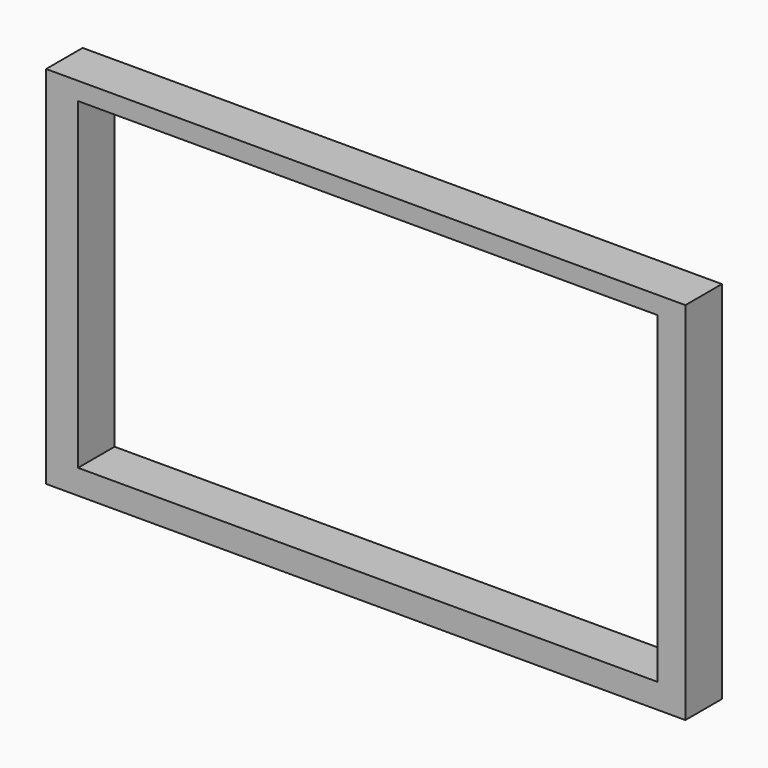
from build123d import *

# Parameters (mm, degrees)
F0_W     = 88.9
F0_H     = 50.8
F0_W_2   = 80.5856101215
F0_H_2   = 44.8976987973
F1_DEPTH = 6.35


# Not quite as in the source:
# - the program builds the solid bodies; features that only make, move or delete a surface that nothing else refers to are left out


with BuildPart() as f1:
    # F0 (on Front) → F1 (new body)
    with BuildSketch(Plane.XZ):
        with Locations((8.7780728936, 7.7330259998)):
            Rectangle(F0_W, F0_H)
        with Locations((9.0658795089, 8.2024647854)):
            Rectangle(F0_W_2, F0_H_2, mode=Mode.SUBTRACT)
    extrude(amount=F1_DEPTH)


solid = f1.part
